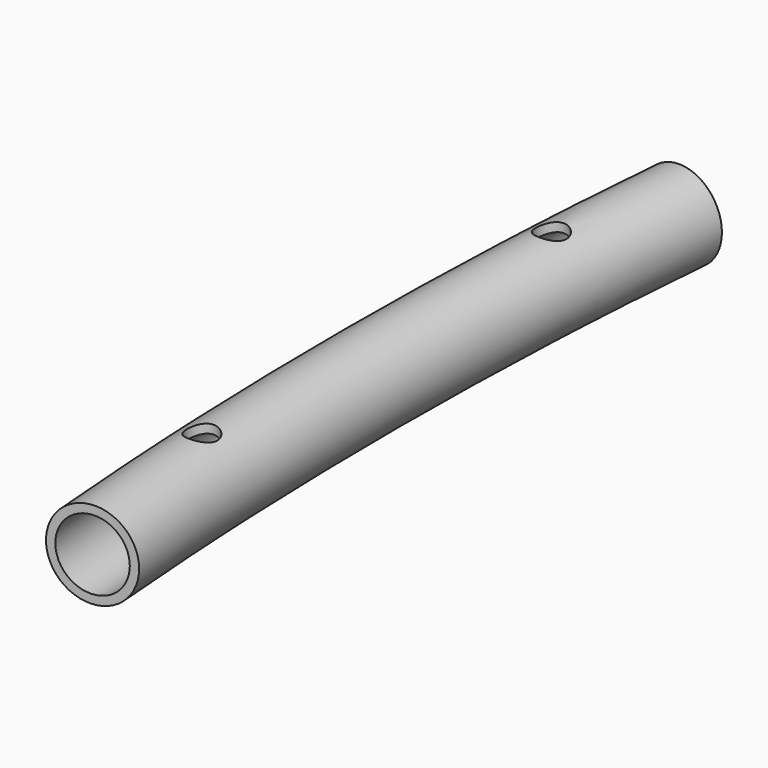
from build123d import *
from build123d import SkipClean  # not in build123d's __all__

# Parameters (mm, degrees)
F0_R          = 15
F0_R_2        = 12
F1_ANGLE_BACK = 5
F1_ANGLE      = 10
F2_R          = 5.25
F3_DEPTH      = 15.001
F3_DEPTH_BACK = 15.001


with BuildPart() as f1:
    # F0 (on Front) → F1 (revolve)
    with BuildSketch(Plane.XZ, mode=Mode.PRIVATE) as f1_sk:
        with Locations((-1450, 0)):
            Circle(F0_R)
        with Locations((-1450, 0)):
            Circle(F0_R_2, mode=Mode.SUBTRACT)
    revolve(f1_sk.sketch.rotate(Axis((0, 0, 190.0846064091), (0, 0, -1)), -F1_ANGLE_BACK), axis=Axis((0, 0, 190.0846064091), (0, 0, -1)), revolution_arc=F1_ANGLE)

    # F2 (on Top) → F3 (cut, two sides)
    with BuildSketch(Plane.XY) as f3_sk:
        with Locations((-1448.0590457575, -75)):
            Circle(F2_R)
        with Locations((-1448.0590457575, 75)):
            Circle(F2_R)
    with SkipClean():  # cleaning this boolean's faces spoils the solid; the shape is the same uncleaned
        extrude(amount=-F3_DEPTH, mode=Mode.SUBTRACT)
        extrude(f3_sk.sketch, amount=F3_DEPTH_BACK, mode=Mode.SUBTRACT)


solid = f1.part
